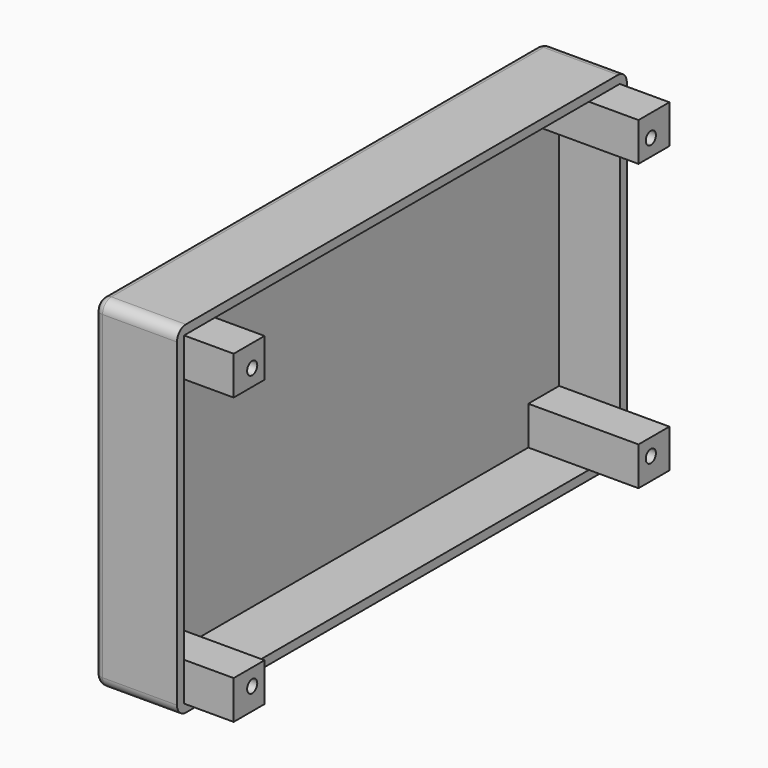
from build123d import *

# Parameters (mm, degrees)
F0_W         = 102
F0_H         = 62
F1_DEPTH     = 15
F2_R         = 1.5
F3_W         = 98.8
F3_H         = 58.8
F4_DEPTH     = 11
F5_W         = 7
F5_H         = 7
F5_R         = 1.15
F6_DEPTH     = 20
F7_T1_DEPTH  = 20
F7_T4_ANGLE  = 90
F7_T6_ANGLE  = 90
F7_T8_ANGLE  = 90
F7_T10_ANGLE = 90


# Not quite as in the source:
# - a fillet or chamfer that OpenCascade refuses, or shapes differently, is made with other operations: its cross-section is extruded or revolved along the edge and cut away or added
# - a feature names something its author has since deleted; it is built from what else it names


with BuildPart() as f1:
    # F0 (on Right) → F1 (new body)
    with BuildSketch(Plane.YZ):
        with Locations((-6.9849695861, 0.5)):
            Rectangle(F0_W, F0_H)
    extrude(amount=-F1_DEPTH)

    # F2
    f2_edges = [f1.edges().sort_by_distance(p)[0] for p in [
        (-15, -6.98497, 31.5),
        (-15, -57.98497, 0.5),
        (-15, -6.98497, -30.5),
        (-15, 44.01503, 0.5),
    ]]
    fillet(f2_edges, radius=F2_R)

    # F3 (on face) → F4 (cut)
    with BuildSketch(Plane.YZ):
        with Locations((-6.9849695861, 0.5)):
            Rectangle(F3_W, F3_H)
    extrude(amount=-F4_DEPTH, mode=Mode.SUBTRACT)

    # F5 (on face) → F6 (join)
    with BuildSketch(Plane.YZ.offset(-11)):
        with Locations((-52.8849695861, -25.4)):
            Rectangle(F5_W, F5_H)
        with Locations((-52.1849695861, -24.9)):
            Circle(F5_R, mode=Mode.SUBTRACT)
        with Locations((38.9150304139, -25.4)):
            Rectangle(F5_W, F5_H)
        with Locations((38.2150304139, -24.9)):
            Circle(F5_R, mode=Mode.SUBTRACT)
        with Locations((38.9150304139, 26.4)):
            Rectangle(F5_W, F5_H)
        with Locations((38.2150304139, 25.9)):
            Circle(F5_R, mode=Mode.SUBTRACT)
        with Locations((-52.8849695861, 26.4)):
            Rectangle(F5_W, F5_H)
        with Locations((-52.1849695861, 25.9)):
            Circle(F5_R, mode=Mode.SUBTRACT)
    extrude(amount=F6_DEPTH)

    # F7: fillet of radius 2 on 4 edges, made by hand

    # F7_s2 → F7_t1 (cut)
    with BuildSketch(Plane.YZ.offset(-15)):
        with BuildLine():
            ThreePointArc((-55.9849695861, -30.5), (-57.3991831485, -29.9142135624), (-57.9849695861, -28.5))
            Line((-57.9849695861, -28.5), (-57.9849695861, -30.5))
            Line((-57.9849695861, -30.5), (-55.9849695861, -30.5))
        make_face()
        with BuildLine():
            ThreePointArc((-57.9849695861, 29.5), (-57.3991831485, 30.9142135624), (-55.9849695861, 31.5))
            Line((-55.9849695861, 31.5), (-57.9849695861, 31.5))
            Line((-57.9849695861, 31.5), (-57.9849695861, 29.5))
        make_face()
        with BuildLine():
            ThreePointArc((44.0150304139, 29.5), (43.4292439762, 30.9142135624), (42.0150304139, 31.5))
            Line((42.0150304139, 31.5), (44.0150304139, 31.5))
            Line((44.0150304139, 31.5), (44.0150304139, 29.5))
        make_face()
        with BuildLine():
            ThreePointArc((42.0150304139, -30.5), (43.4292439762, -29.9142135624), (44.0150304139, -28.5))
            Line((44.0150304139, -28.5), (44.0150304139, -30.5))
            Line((44.0150304139, -30.5), (42.0150304139, -30.5))
        make_face()
    extrude(amount=F7_T1_DEPTH, mode=Mode.SUBTRACT)

    # F7_s3 → F7_t4 (revolve, cut)
    with BuildSketch(Plane.XY.offset(-28.5)):
        with BuildLine():
            ThreePointArc((-15, 42.5150304139), (-14.5606601718, 43.5756905856), (-13.5, 44.0150304139))
            Line((-13.5, 44.0150304139), (-15, 44.0150304139))
            Line((-15, 44.0150304139), (-15, 42.5150304139))
        make_face()
    revolve(axis=Axis((-15, 42.0150304139, -28.5), (-1, 0, 0)), revolution_arc=F7_T4_ANGLE, mode=Mode.SUBTRACT)

    # F7_s5 → F7_t6 (revolve, cut)
    with BuildSketch(Plane.XZ.offset(-42.0150304139)):
        with BuildLine():
            ThreePointArc((-15, 30), (-14.5606601718, 31.0606601718), (-13.5, 31.5))
            Line((-13.5, 31.5), (-15, 31.5))
            Line((-15, 31.5), (-15, 30))
        make_face()
    revolve(axis=Axis((-15, 42.0150304139, 29.5), (-1, 0, 0)), revolution_arc=F7_T6_ANGLE, mode=Mode.SUBTRACT)

    # F7_s7 → F7_t8 (revolve, cut)
    with BuildSketch(Plane.XY.offset(29.5)):
        with BuildLine():
            ThreePointArc((-15, -56.4849695861), (-14.5606601718, -57.5456297579), (-13.5, -57.9849695861))
            Line((-13.5, -57.9849695861), (-15, -57.9849695861))
            Line((-15, -57.9849695861), (-15, -56.4849695861))
        make_face()
    revolve(axis=Axis((-15, -55.9849695861, 29.5), (-1, 0, 0)), revolution_arc=F7_T8_ANGLE, mode=Mode.SUBTRACT)

    # F7_s9 → F7_t10 (revolve, cut)
    with BuildSketch(Plane.XZ.offset(55.9849695861)):
        with BuildLine():
            ThreePointArc((-15, -29), (-14.5606601718, -30.0606601718), (-13.5, -30.5))
            Line((-13.5, -30.5), (-15, -30.5))
            Line((-15, -30.5), (-15, -29))
        make_face()
    revolve(axis=Axis((-15, -55.9849695861, -28.5), (-1, 0, 0)), revolution_arc=F7_T10_ANGLE, mode=Mode.SUBTRACT)


solid = f1.part
